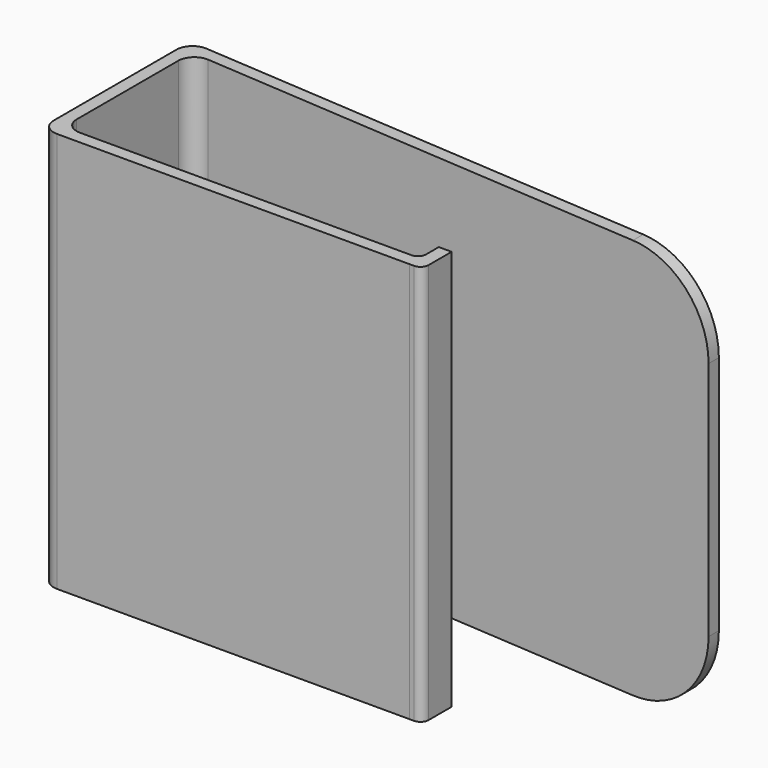
from build123d import *

# Parameters (mm, degrees)
F1_DEPTH = 25
F2_R     = 5
F3_R     = 1
F4_R     = 0.5


# Not quite as in the source:
# - a feature names something its author has since deleted; it is built from what else it names


with BuildPart() as f1:
    # F0 (on Top) → F1 (new body)
    with BuildSketch(Plane.XY):
        Polygon((-12.9449461493, 23.2145217315), (-12.9449461493, 11.7507396201), (10.0550538507, 11.7507396201), (10.8550538507, 11.7466916821), (10.8550538507, 14.0507396201), (10.0550538507, 14.0507396201), (10.0550538507, 12.5507396201), (-12.1449461493, 12.5507396201), (-12.1449461493, 22.5507396201), (22.0030346708, 20.162880187), (22.0030346708, 20.9648337055), (-12.9449461493, 23.4086345881), align=None)
    extrude(amount=F1_DEPTH)

    # F2
    f2_edges = [f1.edges().sort_by_distance(p)[0] for p in [
        (22.003035, 20.563857, 25),
        (22.003035, 20.563857, 0),
    ]]
    fillet(f2_edges, radius=F2_R)

    # F3
    f3_edges = [f1.edges().sort_by_distance(p)[0] for p in [
        (-12.944946, 11.75074, 12.5),
        (-12.144946, 12.55074, 12.5),
        (-12.944946, 23.408635, 12.5),
        (-12.144946, 22.55074, 12.5),
    ]]
    fillet(f3_edges, radius=F3_R)

    # F4
    f4_edges = [f1.edges().sort_by_distance(p)[0] for p in [
        (10.855054, 11.746692, 12.5),
        (10.055054, 12.55074, 12.5),
    ]]
    fillet(f4_edges, radius=F4_R)


solid = f1.part
